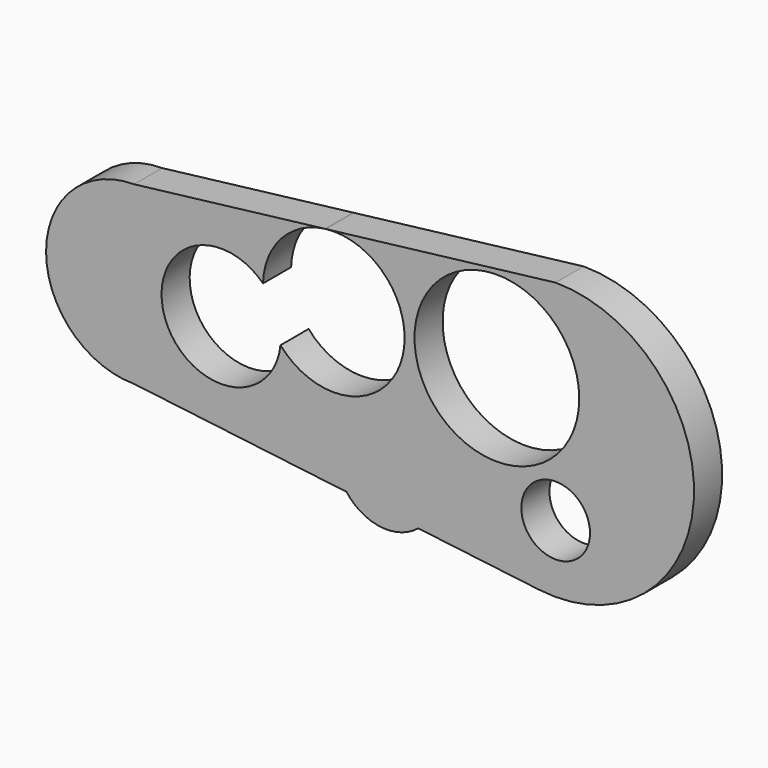
from build123d import *

# Parameters (mm, degrees)
F0_R     = 24.8141888618
F0_R_2   = 59.5346246142
F1_DEPTH = 25.4


with BuildPart() as f1:
    # F0 (on Front) → F1 (new body)
    with BuildSketch(Plane.XZ):
        with BuildLine():
            Line((-99.2976298759, -88.6105044971), (-12.1288724864, -99.2617270261))
            ThreePointArc((-12.1288724864, -99.2617270261), (99.8152611143, -6.0756603504), (0, 100))
            Line((0, 100), (-166.1658385565, 80.1015318002))
            ThreePointArc((-166.1658385565, 80.1015318002), (-126.2736372151, 67.4381308089), (-109.1637541986, 29.2412545532))
            ThreePointArc((-109.1637541986, 29.2412545532), (-142.3543083636, -18.6806916137), (-198.8867849114, -4.4608144844))
            ThreePointArc((-198.8867849114, -4.4608144844), (-282.3141058144, -14.5707555174), (-211.5247269524, 30.7193385549))
            ThreePointArc((-211.5247269524, 30.7193385549), (-198.2429888587, 63.6654948362), (-166.717182755, 80.0355079706))
            Line((-166.717182755, 80.0355079706), (-304.8, 63.5))
            ThreePointArc((-304.8, 63.5), (-368.3, 0), (-304.8, -63.5))
            Line((-304.8, -63.5), (-151.1628675473, -82.2730482283))
            ThreePointArc((-151.1628675473, -82.2730482283), (-133.5991325998, -26.3279382936), (-86.0463709553, -60.6364645064))
            ThreePointArc((-86.0463709553, -60.6364645064), (-89.5267066571, -76.1134052278), (-99.2976298759, -88.6105044971))
        make_face()
        with Locations((0, -51.3095334172)):
            Circle(F0_R, mode=Mode.SUBTRACT)
        with Locations((-42.4963980913, 31.7849628627)):
            Circle(F0_R_2, mode=Mode.SUBTRACT)
        with BuildLine():
            ThreePointArc((-151.1628675473, -82.2730482283), (-126.5842058284, -96.5224536382), (-99.2976298759, -88.6105044971))
            Line((-99.2976298759, -88.6105044971), (-151.1628675473, -82.2730482283))
        make_face()
        with BuildLine():
            Line((-151.1628675473, -82.2730482283), (-99.2976298759, -88.6105044971))
            ThreePointArc((-99.2976298759, -88.6105044971), (-89.5267066571, -76.1134052278), (-86.0463709553, -60.6364645064))
            ThreePointArc((-86.0463709553, -60.6364645064), (-133.5991325998, -26.3279382936), (-151.1628675473, -82.2730482283))
        make_face()
    extrude(amount=F1_DEPTH)


with BuildPart() as f1b:
    # F0 (on Front) → F1, piece 2 (new body)
    with BuildSketch(Plane.XZ):
        with BuildLine():
            Line((-166.717182755, 80.0355079706), (-166.1658385565, 80.1015318002))
            ThreePointArc((-166.1658385565, 80.1015318002), (-166.4416001786, 80.069267462), (-166.717182755, 80.0355079706))
        make_face()
    extrude(amount=F1_DEPTH)


solid = Compound([f1.part, f1b.part])
